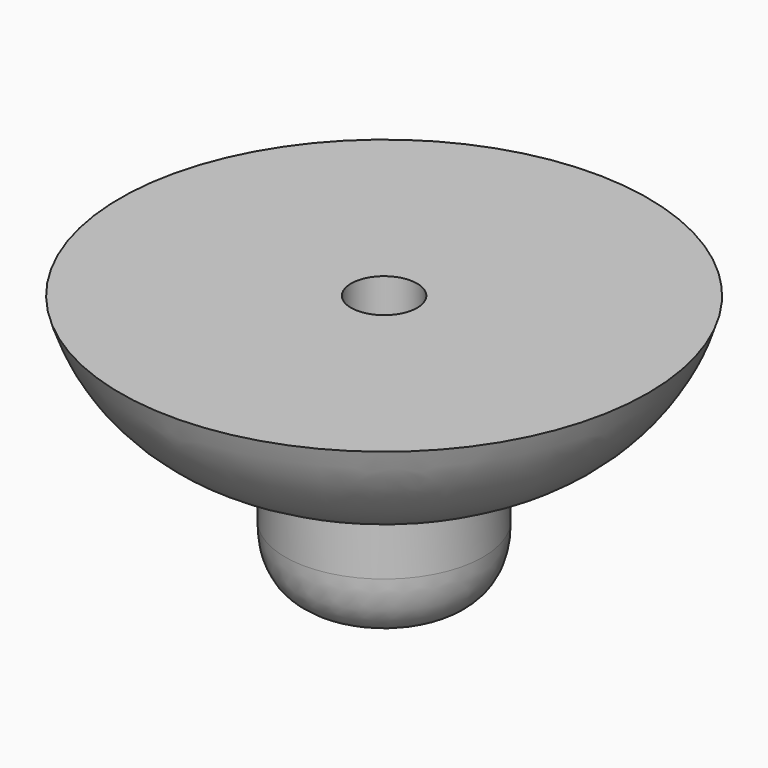
from build123d import *

# Parameters (mm, degrees)
F2_R     = 0.25
F3_DEPTH = 2.001


# Not quite as in the source:
# - a fillet or chamfer that OpenCascade refuses, or shapes differently, is made with other operations: its cross-section is extruded or revolved along the edge and cut away or added


with BuildPart() as f1:
    # F0 (on Front) → F1 (revolve)
    with BuildSketch(Plane.XZ):
        with BuildLine():
            Line((2, 0), (0, 0))
            Line((0, 0), (0, -2))
            Line((0, -2), (0.75, -2))
            Line((0.75, -2), (0.75, -1))
            ThreePointArc((0.75, -1), (1.533581534, -0.6982269175), (2, 0))
        make_face()
    revolve(axis=Axis((0, 0, -1.625075005), (0, 0, -1)))

    # F2 (on face) → F3 (cut, through all)
    with BuildSketch(Plane.XY):
        Circle(F2_R)
    extrude(amount=-F3_DEPTH, mode=Mode.SUBTRACT)

    # F4: fillet of radius 0.5 on 1 edges, made by hand

    # F4_s1 → F4_t2 (revolve, cut)
    with BuildSketch(Plane.XZ):
        with BuildLine():
            add(Edge.make_bspline(
                [(0.75, -1.5), (0.75, -2), (0.25, -2)],
                knots=[0, 0, 0, 1, 1, 1], degree=2, weights=[1, 1, 1]))
            Line((0.25, -2), (0.75, -2))
            Line((0.75, -2), (0.75, -1.5))
        make_face()
    revolve(axis=Axis((0, 0, -2), (0, 0, -1)), mode=Mode.SUBTRACT)


solid = f1.part
